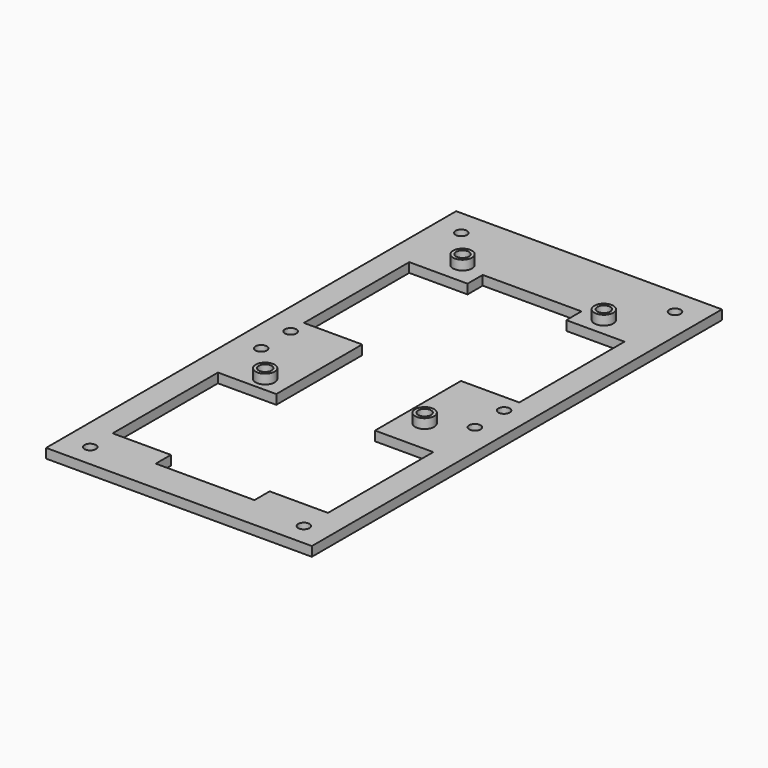
from build123d import *

# Parameters (mm, degrees)
F0_R     = 1.905
F0_R_2   = 3.175
F1_DEPTH = 3.175
F0_R_3   = 2.1456580426
F2_DEPTH = 6.35


# Not quite as in the source:
# - ends of sketch curves that miss each other by under 0.0002 mm in the source are joined


with BuildPart() as f1:
    # F0 (on Top) → F1 (new body)
    with BuildSketch(Plane.XY):
        Polygon((44.45, 44.4739684463), (-44.45, 44.4739684463), (-44.45, -126.9760241032), (44.4500006139, -126.9760241032), align=None)
        with Locations((-35.7399480417, -119.4167938083)):
            Circle(F0_R, mode=Mode.SUBTRACT)
        with Locations((-35.7399480417, -47.9368977249)):
            Circle(F0_R, mode=Mode.SUBTRACT)
        with Locations((-24.13, -60.7800519583)):
            Circle(F0_R_2, mode=Mode.SUBTRACT)
        Polygon((-16.5099999687, 14.3167711779), (-16.5099999992, 20.6667711779), (16.5100000008, 20.6667711779), (16.5100000313, 14.3167711779), (36.0137783311, 14.3167711779), (36.0137783311, -29.7200025995), (16.5100000008, -29.7200026932), (16.5099995171, -65.6599379314), (36.013777817, -65.6599379314), (36.013777817, -109.6967117089), (16.5099994866, -109.6967118025), (16.5099995476, -116.0467118025), (-16.5100004524, -116.0467118025), (-16.5100004829, -109.6967118025), (-36.0137786019, -109.6967118961), (-36.0137788132, -65.659938025), (-16.5100004829, -65.6599379314), (-16.5099999687, -29.7200026932), (-36.0137780877, -29.7200027868), (-36.0137782991, 14.3167710843), align=None, mode=Mode.SUBTRACT)
        with Locations((35.7399480417, -119.4167938083)):
            Circle(F0_R, mode=Mode.SUBTRACT)
        with Locations((24.1312399077, -54.422124289)):
            Circle(F0_R_2, mode=Mode.SUBTRACT)
        with Locations((35.7399480417, -47.9368977249)):
            Circle(F0_R, mode=Mode.SUBTRACT)
        with Locations((-35.7399480417, -35.6178977249)):
            Circle(F0_R, mode=Mode.SUBTRACT)
        with Locations((-24.142025454, 21.7699480417)):
            Circle(F0_R_2, mode=Mode.SUBTRACT)
        with Locations((-35.7399480417, 35.7399480417)):
            Circle(F0_R, mode=Mode.SUBTRACT)
        with Locations((35.7399480417, -35.7399480417)):
            Circle(F0_R, mode=Mode.SUBTRACT)
        with Locations((24.13, 20.4999480417)):
            Circle(F0_R_2, mode=Mode.SUBTRACT)
        with Locations((35.7399480417, 35.7399480417)):
            Circle(F0_R, mode=Mode.SUBTRACT)
    extrude(amount=F1_DEPTH)

    # F0 (on Top) → F2 (join)
    with BuildSketch(Plane.XY):
        with Locations((-24.13, -60.7800519583)):
            Circle(F0_R_2)
        with Locations((-24.13, -60.7800519583)):
            Circle(F0_R_3, mode=Mode.SUBTRACT)
        with Locations((-24.142025454, 21.7699480417)):
            Circle(F0_R_2)
        with Locations((-24.142025454, 21.7699480417)):
            Circle(F0_R_3, mode=Mode.SUBTRACT)
        with Locations((24.1312399077, -54.422124289)):
            Circle(F0_R_2)
        with Locations((24.1312399077, -54.422124289)):
            Circle(F0_R_3, mode=Mode.SUBTRACT)
        with Locations((24.13, 20.4999480417)):
            Circle(F0_R_2)
        with Locations((24.13, 20.4999480417)):
            Circle(F0_R_3, mode=Mode.SUBTRACT)
    extrude(amount=F2_DEPTH)


solid = f1.part
